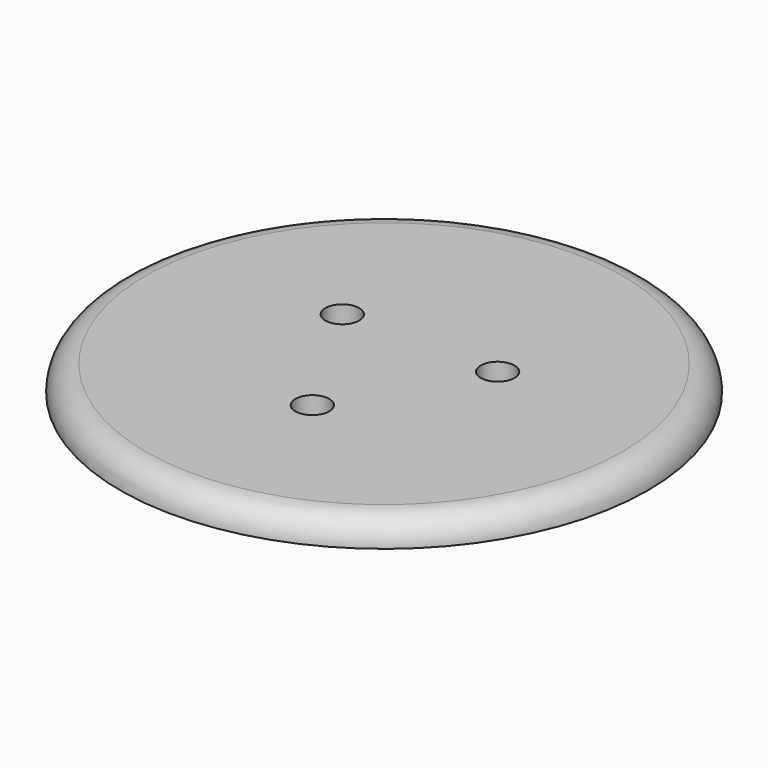
from build123d import *

# Parameters (mm, degrees)
F0_R           = 38.5
F1_DEPTH       = 6.9
F0_R_2         = 51.5
F2_DEPTH       = 5
F4_D           = 6.6
F4_CBORE_D     = 11.25
F4_CBORE_DEPTH = 6
F6_D           = 5.5
F6_DEPTH       = 9
F6_TIP         = 1.6523667023
F7_R           = 4.99999
F8_SIZE        = 1


# Not quite as in the source:
# - a fillet or chamfer is up to 0.001 mm smaller than in the source, because OpenCascade refuses the exact size


with BuildPart() as f1:
    # F0 (on Top) → F1 (new body)
    with BuildSketch(Plane.XY):
        Circle(F0_R)
    extrude(amount=-F1_DEPTH)

    # F0 (on Top) → F2 (join)
    with BuildSketch(Plane.XY):
        Circle(F0_R_2)
        Circle(F0_R, mode=Mode.SUBTRACT)
        Circle(F0_R)
    extrude(amount=F2_DEPTH)

    # F4 (through all)
    with Locations(Plane(origin=(0, 0, -6.9), x_dir=(1, 0, 0), z_dir=(0, 0, -1))):
        with Locations((-15.1554445662, -8.75), (0, 17.5), (15.1554445662, -8.75)):
            CounterBoreHole(F4_D / 2, F4_CBORE_D / 2, F4_CBORE_DEPTH)

    # F6
    with Locations(Plane(origin=(0, 0, -6.9), x_dir=(1, 0, 0), z_dir=(0, 0, -1))):
        with Locations((-12, 0), (12, 0)):
            Hole(F6_D / 2, depth=F6_DEPTH)
            with Locations((0, 0, -(F6_DEPTH + F6_TIP / 2))):  # 118° drill point
                Cone(0, F6_D / 2, F6_TIP, mode=Mode.SUBTRACT)

    # F7 (radius 5 in the source; OpenCascade refuses exactly that, so slightly less here)
    f7_edges = [f1.edges().sort_by_distance(p)[0] for p in [
        (-51.5, 0, 5),
    ]]
    fillet(f7_edges, radius=F7_R)

    # F8
    f8_edges = [f1.edges().sort_by_distance(p)[0] for p in [
        (-38.5, 0, -6.9),
    ]]
    chamfer(f8_edges, length=F8_SIZE)


solid = f1.part
